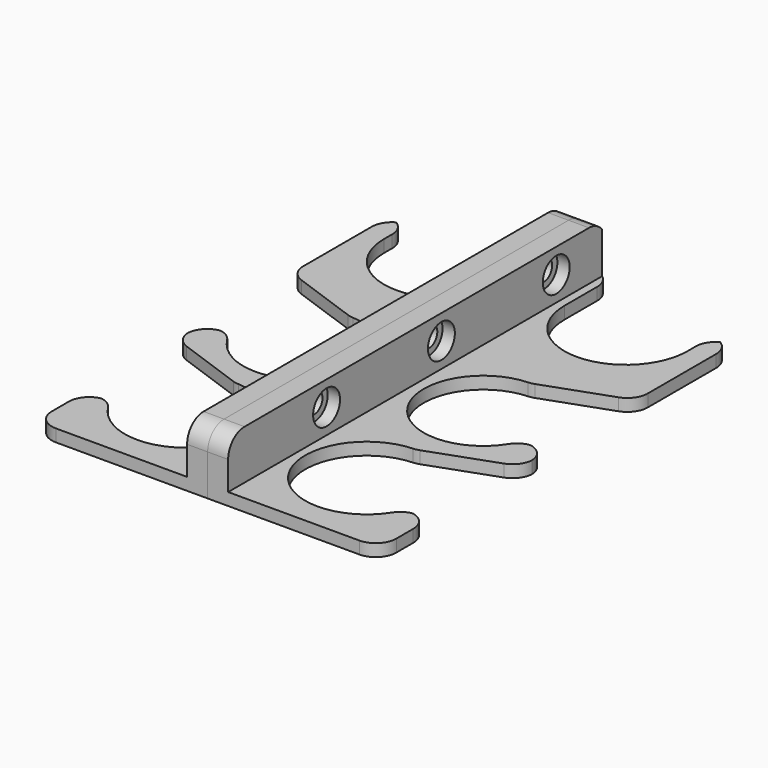
from build123d import *

# Parameters (mm, degrees)
F1_DEPTH     = 3
F0_W         = 5
F0_H         = 115
F2_DEPTH     = 15
F3_R         = 4.1
F3_R_2       = 2.5
F4_DEPTH     = 3
F5_DEPTH     = 25
F7_T1_DEPTH  = 28
F7_T3_DEPTH  = 20.6220671379
F7_T5_DEPTH  = 20.5982428035
F7_T7_DEPTH  = 18.234388136
F7_T9_DEPTH  = 17.9629877086
F7_T11_DEPTH = 7.0239301021
F7_T13_DEPTH = 6.9993570631
F7_T15_DEPTH = 30
F8_T1_DEPTH  = 30
F8_T3_DEPTH  = 28
F8_T5_DEPTH  = 20.5982428035
F8_T7_DEPTH  = 20.6220671379
F8_T9_DEPTH  = 6.9993570631
F8_T11_DEPTH = 7.0239301021
F8_T13_DEPTH = 17.9629877086
F8_T15_DEPTH = 18.234388136


# Not quite as in the source:
# - a fillet or chamfer that OpenCascade refuses, or shapes differently, is made with other operations: its cross-section is extruded or revolved along the edge and cut away or added


with BuildPart() as f1:
    # F0 (on Top) → F1 (new body)
    with BuildSketch(Plane.XY):
        with BuildLine():
            Line((7, 0), (5, 0))
            Line((5, 0), (5, -115))
            Line((5, -115), (42, -115))
            Line((42, -115), (42, -99.8333333333))
            Line((42, -99.8333333333), (35.8192699598, -99.8333333333))
            ThreePointArc((35.8192699598, -99.8333333333), (9.5, -102.2915619759), (22, -79))
            Line((22, -79), (42, -71.8333333333))
            Line((42, -71.8333333333), (42, -63.8620689655))
            Line((42, -63.8620689655), (35.4721273899, -63.8620689655))
            ThreePointArc((35.4721273899, -63.8620689655), (10, -66.639410298), (22, -44))
            Line((22, -44), (42, -36.8620689655))
            Line((42, -36.8620689655), (42, -7.5))
            Line((42, -7.5), (37, -7.5))
            Line((37, -7.5), (37, -15))
            ThreePointArc((37, -15), (22, -30), (7, -15))
            Line((7, -15), (7, 0))
        make_face()
    extrude(amount=F1_DEPTH)

    # F0 (on Top) → F2 (join)
    with BuildSketch(Plane.XY):
        with Locations((2.5, -57.5)):
            Rectangle(F0_W, F0_H)
    extrude(amount=F2_DEPTH)

    # F3 (on face) → F4 (cut)
    with BuildSketch(Plane.YZ.offset(5)):
        with Locations((-85, 9)):
            Circle(F3_R)
        with Locations((-85, 9)):
            Circle(F3_R_2, mode=Mode.SUBTRACT)
        with Locations((-50, 9)):
            Circle(F3_R)
        with Locations((-50, 9)):
            Circle(F3_R_2, mode=Mode.SUBTRACT)
        with Locations((-15, 9)):
            Circle(F3_R)
        with Locations((-15, 9)):
            Circle(F3_R_2, mode=Mode.SUBTRACT)
    extrude(amount=-F4_DEPTH, mode=Mode.SUBTRACT)

    # F5 (cut): faces of the model
    f5_faces = [f1.faces().sort_by_distance(p)[0] for p in [
        (5, -15, 9),
        (5, -50, 9),
        (5, -85, 9),
    ]]
    extrude(f5_faces, amount=-F5_DEPTH, mode=Mode.SUBTRACT)


with BuildPart() as f6_1:
    # F6: instance of F1
    add(f1.part.mirror(Plane(origin=(0, -57.7651628091, 7.4469674382), x_dir=(0, -1, 0), z_dir=(-1, 0, 0))))

    # F7: fillet of radius 5 on 14 edges, made by hand

    # F7_s2 → F7_t1 (cut)
    with BuildSketch(Plane.XY.offset(-12.5)):
        with BuildLine():
            ThreePointArc((-37, -115), (-40.5355339059, -113.5355339059), (-42, -110))
            Line((-42, -110), (-42, -115))
            Line((-42, -115), (-37, -115))
        make_face()
        with BuildLine():
            ThreePointArc((-42, -12.5), (-40.5355339059, -8.9644660941), (-37, -7.5))
            Line((-37, -7.5), (-42, -7.5))
            Line((-42, -7.5), (-42, -12.5))
        make_face()
        with BuildLine():
            ThreePointArc((-42, -7.5), (-38.4644660941, -8.9644660941), (-37, -12.5))
            Line((-37, -12.5), (-37, -7.5))
            Line((-37, -7.5), (-42, -7.5))
        make_face()
        with BuildLine():
            ThreePointArc((-42, -104.8333333333), (-40.5355339059, -101.2977994274), (-37, -99.8333333333))
            Line((-37, -99.8333333333), (-42, -99.8333333333))
            Line((-42, -99.8333333333), (-42, -104.8333333333))
        make_face()
        with BuildLine():
            ThreePointArc((-37, -63.8620689655), (-40.5355339059, -65.3265350596), (-42, -68.8620689655))
            Line((-42, -68.8620689655), (-42, -63.8620689655))
            Line((-42, -63.8620689655), (-37, -63.8620689655))
        make_face()
        with BuildLine():
            ThreePointArc((-7, -5), (-5.5355339059, -1.4644660941), (-2, 0))
            Line((-2, 0), (-7, 0))
            Line((-7, 0), (-7, -5))
        make_face()
    extrude(amount=F7_T1_DEPTH, mode=Mode.SUBTRACT)

    # F7_s4 → F7_t3 (cut)
    with BuildSketch(Plane.XY.offset(-8.8110335689)):
        with BuildLine():
            ThreePointArc((-38.6806532809, -38.0467323636), (-41.0867631693, -36.2183441358), (-42, -33.3376555379))
            Line((-42, -33.3376555379), (-42, -36.8620689655))
            Line((-42, -36.8620689655), (-38.6806532809, -38.0467323636))
        make_face()
    extrude(amount=F7_T3_DEPTH, mode=Mode.SUBTRACT)

    # F7_s6 → F7_t5 (cut)
    with BuildSketch(Plane.XY.offset(-8.7991214017)):
        with BuildLine():
            ThreePointArc((-42, -68.3136847726), (-41.0885971494, -71.191769787), (-38.6866506599, -73.0206168469))
            Line((-38.6866506599, -73.0206168469), (-42, -71.8333333333))
            Line((-42, -71.8333333333), (-42, -68.3136847726))
        make_face()
    extrude(amount=F7_T5_DEPTH, mode=Mode.SUBTRACT)

    # F7_s8 → F7_t7 (cut)
    with BuildSketch(Plane.XY.offset(-7.617194068)):
        with BuildLine():
            ThreePointArc((-34.283362705, -66.2051282051), (-36.0987471591, -64.4868716099), (-38.5190050171, -63.8620689655))
            Line((-38.5190050171, -63.8620689655), (-35.4721273899, -63.8620689655))
            ThreePointArc((-35.4721273899, -63.8620689655), (-34.9309241416, -65.060579307), (-34.283362705, -66.2051282051))
        make_face()
    extrude(amount=F7_T7_DEPTH, mode=Mode.SUBTRACT)

    # F7_s10 → F7_t9 (cut)
    with BuildSketch(Plane.XY.offset(-7.4814938543)):
        with BuildLine():
            ThreePointArc((-38.8118675015, -99.8333333333), (-36.4182997321, -100.443477603), (-34.6089006261, -102.125))
            ThreePointArc((-34.6089006261, -102.125), (-35.2636715942, -101.0053562252), (-35.8192699598, -99.8333333333))
            Line((-35.8192699598, -99.8333333333), (-38.8118675015, -99.8333333333))
        make_face()
    extrude(amount=F7_T9_DEPTH, mode=Mode.SUBTRACT)

    # F7_s12 → F7_t11 (cut)
    with BuildSketch(Plane.XY.offset(-2.011965051)):
        with BuildLine():
            ThreePointArc((-21.3032229749, -79.0161920135), (-22.0411403271, -78.9265621167), (-22.7576146265, -78.7285214255))
            Line((-22.7576146265, -78.7285214255), (-22, -79))
            ThreePointArc((-22, -79), (-21.6515174309, -79.0040485497), (-21.3032229749, -79.0161920135))
        make_face()
    extrude(amount=F7_T11_DEPTH, mode=Mode.SUBTRACT)

    # F7_s14 → F7_t13 (cut)
    with BuildSketch(Plane.XY.offset(-1.9996785315)):
        with BuildLine():
            ThreePointArc((-21.3104528016, -44.0164049815), (-22.0424386394, -43.9271168274), (-22.7533311865, -43.7311386972))
            Line((-22.7533311865, -43.7311386972), (-22, -44))
            ThreePointArc((-22, -44), (-21.6551288421, -44.0041018255), (-21.3104528016, -44.0164049815))
        make_face()
    extrude(amount=F7_T13_DEPTH, mode=Mode.SUBTRACT)

    # F7_s16 → F7_t15 (cut)
    with BuildSketch(Plane.YZ.offset(-17.5)):
        with BuildLine():
            ThreePointArc((0, 10), (-1.4644660941, 13.5355339059), (-5, 15))
            Line((-5, 15), (0, 15))
            Line((0, 15), (0, 10))
        make_face()
        with BuildLine():
            ThreePointArc((-115, 10), (-113.5355339059, 13.5355339059), (-110, 15))
            Line((-110, 15), (-115, 15))
            Line((-115, 15), (-115, 10))
        make_face()
    extrude(amount=F7_T15_DEPTH, mode=Mode.SUBTRACT)


with BuildPart() as f1_1:
    add(f1.part)

    # F8: fillet of radius 5 on 14 edges, made by hand

    # F8_s2 → F8_t1 (cut)
    with BuildSketch(Plane.YZ.offset(-12.5)):
        with BuildLine():
            ThreePointArc((-115, 10), (-113.5355339059, 13.5355339059), (-110, 15))
            Line((-110, 15), (-115, 15))
            Line((-115, 15), (-115, 10))
        make_face()
        with BuildLine():
            ThreePointArc((0, 10), (-1.4644660941, 13.5355339059), (-5, 15))
            Line((-5, 15), (0, 15))
            Line((0, 15), (0, 10))
        make_face()
    extrude(amount=F8_T1_DEPTH, mode=Mode.SUBTRACT)

    # F8_s4 → F8_t3 (cut)
    with BuildSketch(Plane.XY.offset(-12.5)):
        with BuildLine():
            ThreePointArc((37, -115), (40.5355339059, -113.5355339059), (42, -110))
            Line((42, -110), (42, -115))
            Line((42, -115), (37, -115))
        make_face()
        with BuildLine():
            ThreePointArc((42, -104.8333333333), (40.5355339059, -101.2977994274), (37, -99.8333333333))
            Line((37, -99.8333333333), (42, -99.8333333333))
            Line((42, -99.8333333333), (42, -104.8333333333))
        make_face()
        with BuildLine():
            ThreePointArc((37, -63.8620689655), (40.5355339059, -65.3265350596), (42, -68.8620689655))
            Line((42, -68.8620689655), (42, -63.8620689655))
            Line((42, -63.8620689655), (37, -63.8620689655))
        make_face()
        with BuildLine():
            ThreePointArc((42, -7.5), (38.4644660941, -8.9644660941), (37, -12.5))
            Line((37, -12.5), (37, -7.5))
            Line((37, -7.5), (42, -7.5))
        make_face()
        with BuildLine():
            ThreePointArc((42, -12.5), (40.5355339059, -8.9644660941), (37, -7.5))
            Line((37, -7.5), (42, -7.5))
            Line((42, -7.5), (42, -12.5))
        make_face()
        with BuildLine():
            ThreePointArc((7, -5), (5.5355339059, -1.4644660941), (2, 0))
            Line((2, 0), (7, 0))
            Line((7, 0), (7, -5))
        make_face()
    extrude(amount=F8_T3_DEPTH, mode=Mode.SUBTRACT)

    # F8_s6 → F8_t5 (cut)
    with BuildSketch(Plane.XY.offset(-8.7991214017)):
        with BuildLine():
            ThreePointArc((42, -68.3136847726), (41.0885971494, -71.191769787), (38.6866506599, -73.0206168469))
            Line((38.6866506599, -73.0206168469), (42, -71.8333333333))
            Line((42, -71.8333333333), (42, -68.3136847726))
        make_face()
    extrude(amount=F8_T5_DEPTH, mode=Mode.SUBTRACT)

    # F8_s8 → F8_t7 (cut)
    with BuildSketch(Plane.XY.offset(-8.8110335689)):
        with BuildLine():
            ThreePointArc((38.6806532809, -38.0467323636), (41.0867631693, -36.2183441358), (42, -33.3376555379))
            Line((42, -33.3376555379), (42, -36.8620689655))
            Line((42, -36.8620689655), (38.6806532809, -38.0467323636))
        make_face()
    extrude(amount=F8_T7_DEPTH, mode=Mode.SUBTRACT)

    # F8_s10 → F8_t9 (cut)
    with BuildSketch(Plane.XY.offset(-1.9996785315)):
        with BuildLine():
            ThreePointArc((21.3104528016, -44.0164049815), (22.0424386394, -43.9271168274), (22.7533311865, -43.7311386972))
            Line((22.7533311865, -43.7311386972), (22, -44))
            ThreePointArc((22, -44), (21.6551288421, -44.0041018255), (21.3104528016, -44.0164049815))
        make_face()
    extrude(amount=F8_T9_DEPTH, mode=Mode.SUBTRACT)

    # F8_s12 → F8_t11 (cut)
    with BuildSketch(Plane.XY.offset(-2.011965051)):
        with BuildLine():
            ThreePointArc((21.3032229749, -79.0161920135), (22.0411403271, -78.9265621167), (22.7576146265, -78.7285214255))
            Line((22.7576146265, -78.7285214255), (22, -79))
            ThreePointArc((22, -79), (21.6515174309, -79.0040485497), (21.3032229749, -79.0161920135))
        make_face()
    extrude(amount=F8_T11_DEPTH, mode=Mode.SUBTRACT)

    # F8_s14 → F8_t13 (cut)
    with BuildSketch(Plane.XY.offset(-7.4814938543)):
        with BuildLine():
            ThreePointArc((38.8118675015, -99.8333333333), (36.4182997321, -100.443477603), (34.6089006261, -102.125))
            ThreePointArc((34.6089006261, -102.125), (35.2636715942, -101.0053562252), (35.8192699598, -99.8333333333))
            Line((35.8192699598, -99.8333333333), (38.8118675015, -99.8333333333))
        make_face()
    extrude(amount=F8_T13_DEPTH, mode=Mode.SUBTRACT)

    # F8_s16 → F8_t15 (cut)
    with BuildSketch(Plane.XY.offset(-7.617194068)):
        with BuildLine():
            ThreePointArc((34.283362705, -66.2051282051), (36.0987471591, -64.4868716099), (38.5190050171, -63.8620689655))
            Line((38.5190050171, -63.8620689655), (35.4721273899, -63.8620689655))
            ThreePointArc((35.4721273899, -63.8620689655), (34.9309241416, -65.060579307), (34.283362705, -66.2051282051))
        make_face()
    extrude(amount=F8_T15_DEPTH, mode=Mode.SUBTRACT)


solid = Compound([f6_1.part, f1_1.part])
